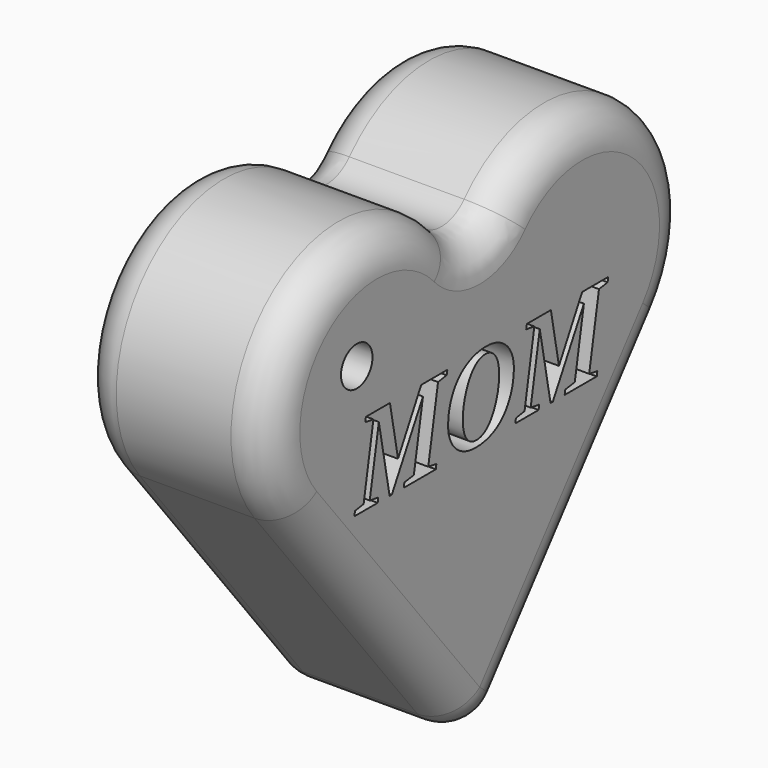
from build123d import *

# Parameters (mm, degrees)
F1_DEPTH     = 25.4
F2_TEXT_SIZE = 16.5817832713
F3_DEPTH     = 152.4
F4_F1_R      = 5.08
F4_F2_R      = 5.08
F5_R         = 2.6170235765
F6_DEPTH     = 152.4


# Not quite as in the source:
# - Text() gives the source's letters only with a copy of the font that has no kerning and outlines rounded to 1/6400 em; it was checked with that copy


with BuildPart() as f1:
    # F0 (on Right) → F1 (new body)
    with BuildSketch(Plane.YZ):
        with BuildLine():
            Line((-31.0266073793, 0), (0, -38.8684943318))
            Line((0, -38.8684943318), (31.0266073793, 0))
            ThreePointArc((31.0266073793, 0), (25.481787722, 26.9361923073), (0, 16.5929831564))
            ThreePointArc((0, 16.5929831564), (-25.481787722, 26.9361923073), (-31.0266073793, 0))
        make_face()
    extrude(amount=F1_DEPTH)

    # F2 (on face) → F3 (cut)
    with BuildSketch(Plane.YZ.offset(25.4)):
        with Locations((-20.5740000635, -2.2860001773)):
            Text('MOM', F2_TEXT_SIZE, font='Tinos', font_style=FontStyle.BOLDITALIC, text_align=(TextAlign.LEFT, TextAlign.BOTTOM))
    extrude(amount=-F3_DEPTH, mode=Mode.SUBTRACT)

    # F4: fillet of radius 5.08 on 5 edges, made by hand

    # F4_f1
    f4_f1_edges = [f1.edges().sort_by_distance(p)[0] for p in [
        (12.7, 0, 16.5929831564),
    ]]
    fillet(f4_f1_edges, radius=F4_F1_R)

    # F4_f2
    f4_f2_edges = [f1.edges().sort_by_distance(p)[0] for p in [
        (0, 28.6268169067, 24.7954921074),
        (25.4, 28.6268169067, 24.7954921074),
        (12.7, 0, -38.8684943318),
        (25.4, 15.5133036897, -19.4342471659),
        (0, 15.5133036897, -19.4342471659),
        (25.4, 0, 21.4779801589),
        (0, 0, 21.4779801589),
    ]]
    fillet(f4_f2_edges, radius=F4_F2_R)

    # F5 (on face) → F6 (cut)
    with BuildSketch(Plane.YZ.offset(25.4)):
        with Locations((-20.40335536, 15.1090240106)):
            Circle(F5_R)
    extrude(amount=-F6_DEPTH, mode=Mode.SUBTRACT)


solid = f1.part
